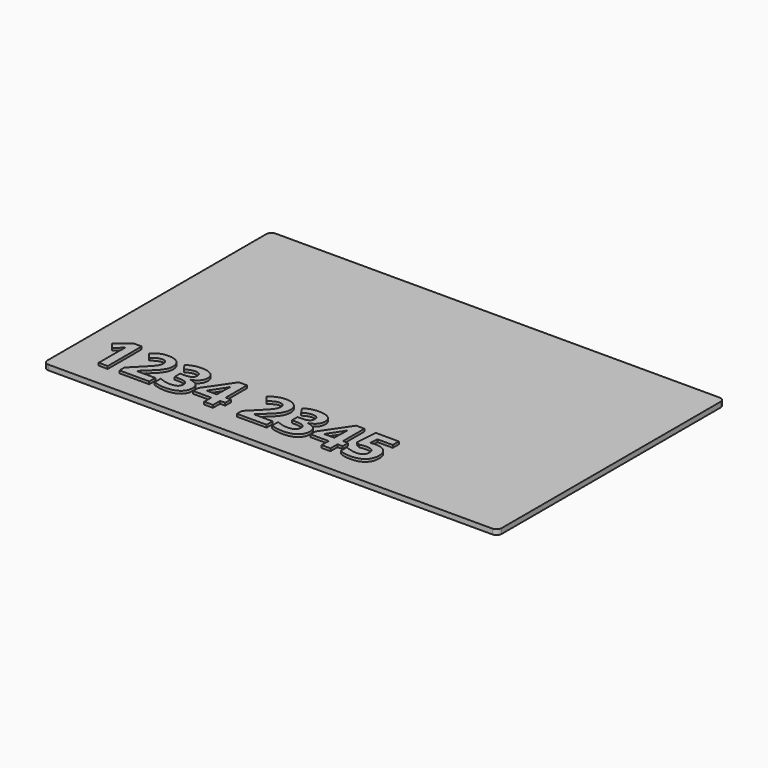
from build123d import *

# Parameters (mm, degrees)
F1_DEPTH     = 1
F2_TEXT_SIZE = 11.536213828
F3_DEPTH     = 0.5


# Not quite as in the source:
# - Text() gives the source's letters only with a copy of the font that has no kerning and outlines rounded to 1/6400 em; it was checked with that copy


with BuildPart() as f1:
    # F0 (on Top) → F1 (new body)
    with BuildSketch(Plane.XY):
        with BuildLine():
            Line((-43, -27.5), (43, -27.5))
            ThreePointArc((43, -27.5), (43.7071067812, -27.2071067812), (44, -26.5))
            Line((44, -26.5), (44, 26.5))
            ThreePointArc((44, 26.5), (43.7071067812, 27.2071067812), (43, 27.5))
            Line((43, 27.5), (-43, 27.5))
            ThreePointArc((-43, 27.5), (-43.7071067812, 27.2071067812), (-44, 26.5))
            Line((-44, 26.5), (-44, -26.5))
            ThreePointArc((-44, -26.5), (-43.7071067812, -27.2071067812), (-43, -27.5))
        make_face()
    extrude(amount=F1_DEPTH)

    # F2 (on face) → F3 (join)
    with BuildSketch(Plane.XY.offset(1)):
        with Locations((-39.8812531494, -23.0214518961)):
            Text('1234 2345', F2_TEXT_SIZE, font='Open Sans', font_style=FontStyle.BOLD, text_align=(TextAlign.LEFT, TextAlign.BOTTOM))
    extrude(amount=F3_DEPTH)


solid = f1.part
